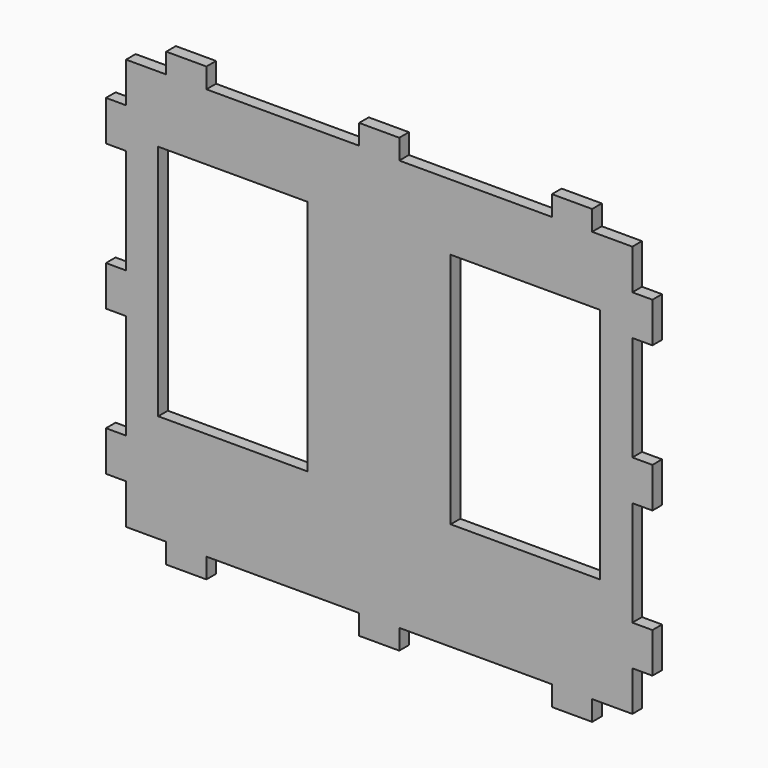
from build123d import *

# Parameters (mm, degrees)
F0_W     = 6.35
F0_H     = 12.7
F0_W_2   = 47.2488999367
F0_H_2   = 75
F0_W_3   = 12.7
F0_H_3   = 6.35
F1_DEPTH = 3.81


# Not quite as in the source:
# - a feature names something its author has since deleted; it is built from what else it names


with BuildPart() as f1:
    # F0 (on Front) → F1 (new body)
    with BuildSketch(Plane.XZ):
        with Locations((-354.6769669852, 49.3793434303)):
            Rectangle(F0_W, F0_H)
        with Locations((-361.0269669852, 49.3793434303)):
            Rectangle(F0_W, F0_H)
        Polygon((-332.4519669852, -61.5706565697), (-284.2019669852, -61.5706565697), (-284.2019669852, -55.2206565697), (-277.8519669852, -55.2206565697), (-277.8519669852, 62.0793434303), (-284.2019669852, 62.0793434303), (-284.2019669852, 68.4293434303), (-332.4519669852, 68.4293434303), (-332.4519669852, 62.0793434303), (-345.1519669852, 62.0793434303), (-345.1519669852, 68.4293434303), (-357.8519669852, 68.4293434303), (-357.8519669852, 55.7293434303), (-351.5019669852, 55.7293434303), (-351.5019669852, 43.0293434303), (-357.8519669852, 43.0293434303), (-357.8519669852, 9.7793434303), (-351.5019669852, 9.7793434303), (-351.5019669852, -2.9206565697), (-357.8519669852, -2.9206565697), (-357.8519669852, -36.1706565697), (-351.5019669852, -36.1706565697), (-351.5019669852, -48.8706565697), (-357.8519669852, -48.8706565697), (-357.8519669852, -61.5706565697), (-345.1519669852, -61.5706565697), (-345.1519669852, -55.2206565697), (-332.4519669852, -55.2206565697), align=None)
        with Locations((-324.0675170169, 10.0176490168)):
            Rectangle(F0_W_2, F0_H_2, mode=Mode.SUBTRACT)
        with Locations((-338.8019669852, 65.2543434303)):
            Rectangle(F0_W_3, F0_H_3)
        with Locations((-338.8019669852, 71.6043434303)):
            Rectangle(F0_W_3, F0_H_3)
        Polygon((-210.5519669852, -61.5706565697), (-197.8519669852, -61.5706565697), (-197.8519669852, -48.8706565697), (-204.2019669852, -48.8706565697), (-204.2019669852, -36.1706565697), (-197.8519669852, -36.1706565697), (-197.8519669852, -2.9206565697), (-204.2019669852, -2.9206565697), (-204.2019669852, 9.7793434303), (-197.8519669852, 9.7793434303), (-197.8519669852, 43.0293434303), (-204.2019669852, 43.0293434303), (-204.2019669852, 55.7293434303), (-197.8519669852, 55.7293434303), (-197.8519669852, 68.4293434303), (-210.5519669852, 68.4293434303), (-210.5519669852, 62.0793434303), (-223.2519669852, 62.0793434303), (-223.2519669852, 68.4293434303), (-271.5019669852, 68.4293434303), (-271.5019669852, 62.0793434303), (-277.8519669852, 62.0793434303), (-277.8519669852, -55.2206565697), (-271.5019669852, -55.2206565697), (-271.5019669852, -61.5706565697), (-223.2519669852, -61.5706565697), (-223.2519669852, -55.2206565697), (-210.5519669852, -55.2206565697), align=None)
        with Locations((-231.6364169536, 10.0176490168)):
            Rectangle(F0_W_2, F0_H_2, mode=Mode.SUBTRACT)
        Polygon((-284.2019669852, 68.4293434303), (-277.8519669852, 68.4293434303), (-271.5019669852, 68.4293434303), (-271.5019669852, 74.7793434303), (-284.2019669852, 74.7793434303), align=None)
        with Locations((-274.6769669852, 65.2543434303)):
            Rectangle(F0_W, F0_H_3)
        with Locations((-281.0269669852, 65.2543434303)):
            Rectangle(F0_W, F0_H_3)
        with Locations((-216.9019669852, 71.6043434303)):
            Rectangle(F0_W_3, F0_H_3)
        with Locations((-216.9019669852, 65.2543434303)):
            Rectangle(F0_W_3, F0_H_3)
        with Locations((-354.6769669852, 3.4293434303)):
            Rectangle(F0_W, F0_H)
        with Locations((-361.0269669852, 3.4293434303)):
            Rectangle(F0_W, F0_H)
        with Locations((-361.0269669852, -42.5206565697)):
            Rectangle(F0_W, F0_H)
        with Locations((-338.8019669852, -64.7456565697)):
            Rectangle(F0_W_3, F0_H_3)
        with Locations((-354.6769669852, -42.5206565697)):
            Rectangle(F0_W, F0_H)
        with Locations((-338.8019669852, -58.3956565697)):
            Rectangle(F0_W_3, F0_H_3)
        with Locations((-281.0269669852, -58.3956565697)):
            Rectangle(F0_W, F0_H_3)
        with Locations((-274.6769669852, -58.3956565697)):
            Rectangle(F0_W, F0_H_3)
        Polygon((-271.5019669852, -67.9206565697), (-271.5019669852, -61.5706565697), (-277.8519669852, -61.5706565697), (-284.2019669852, -61.5706565697), (-284.2019669852, -67.9206565697), align=None)
        with Locations((-216.9019669852, -64.7456565697)):
            Rectangle(F0_W_3, F0_H_3)
        with Locations((-216.9019669852, -58.3956565697)):
            Rectangle(F0_W_3, F0_H_3)
        with Locations((-201.0269669852, -42.5206565697)):
            Rectangle(F0_W, F0_H)
        with Locations((-194.6769669852, -42.5206565697)):
            Rectangle(F0_W, F0_H)
        with Locations((-201.0269669852, 3.4293434303)):
            Rectangle(F0_W, F0_H)
        with Locations((-194.6769669852, 3.4293434303)):
            Rectangle(F0_W, F0_H)
        with Locations((-201.0269669852, 49.3793434303)):
            Rectangle(F0_W, F0_H)
        with Locations((-194.6769669852, 49.3793434303)):
            Rectangle(F0_W, F0_H)
    extrude(amount=F1_DEPTH)


solid = f1.part
